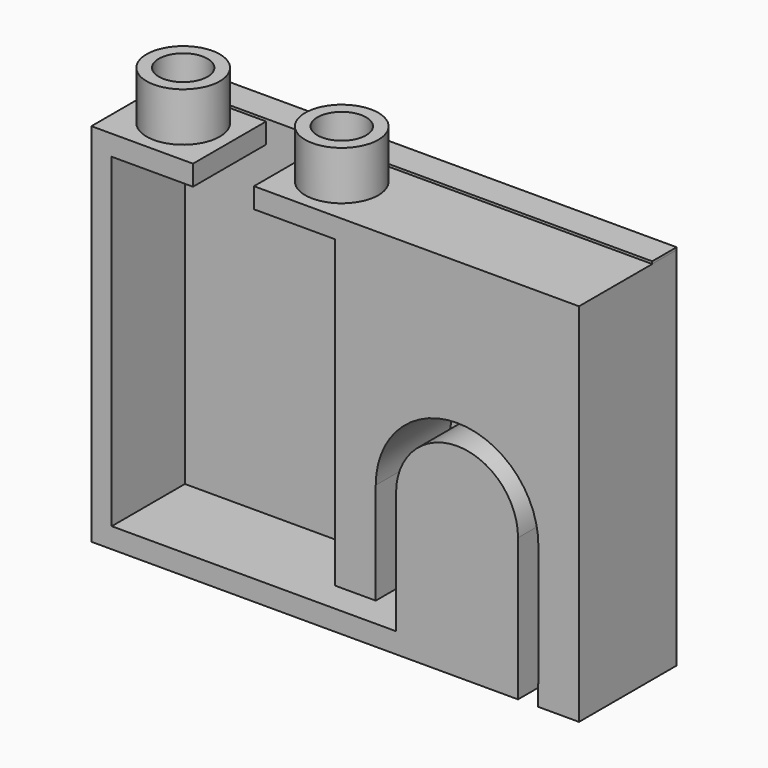
from build123d import *

# Parameters (mm, degrees)
F1_DEPTH = 15.875
F0_W     = 2.6458333332
F0_H     = 42.3358732487
F2_W     = 63.5
F2_H     = 47.625
F2_R     = 3.175
F3_DEPTH = 3.96875
F4_DEPTH = 6.35
F5_R     = 4.7625
F5_R_2   = 3.175
F6_DEPTH = 6.35
F7_R     = 3.175
F8_DEPTH = 25.4


# Not quite as in the source:
# - a feature names something its author has since deleted; it is built from what else it names


with BuildPart() as f1:
    # F0 (on Front) → F1 (new body)
    with BuildSketch(Plane.XZ):
        with BuildLine():
            Line((0, 44.979166582), (-31.75, 44.979166582))
            Line((-31.75, 44.979166582), (-31.75, 42.3358732487))
            Line((-31.75, 42.3358732487), (-31.75, 2.6458333332))
            Line((-31.75, 2.6458333332), (-26.4583333333, 2.6458333332))
            Line((-26.4583333333, 2.6458333332), (-26.4583333333, 15.875))
            ThreePointArc((-26.4583333333, 15.875), (-15.875, 26.4583333333), (-5.2916666667, 15.875))
            Line((-5.2916666667, 15.875), (-5.2916666667, 0))
            Line((-5.2916666667, 0), (0, 0))
            Line((0, 0), (0, 44.979166582))
        make_face()
        Polygon((0, -2.6458333333), (0, 0), (-5.2916666667, 0), (-5.309548229, 0), (-5.309548229, -2.6458333333), align=None)
        Polygon((-31.75, 42.3358732487), (-31.75, 44.979166582), (-34.3958333316, 44.979166582), (-37.0416664956, 44.979166582), (-42.3110765377, 44.979166582), (-42.3110765377, 42.3358732487), (-37.0416664956, 42.3358732487), (-34.3958333316, 42.3358732487), align=None)
    extrude(amount=F1_DEPTH)


with BuildPart() as f1b:
    # F0 (on Front) → F1, piece 2 (new body)
    with BuildSketch(Plane.XZ):
        with BuildLine():
            Line((-23.8125, 0), (-7.9375, 0))
            Line((-7.9375, 0), (-7.9375, 15.875))
            ThreePointArc((-7.9375, 15.875), (-15.875, 23.8125), (-23.8125, 15.875))
            Line((-23.8125, 15.875), (-23.8125, 0))
        make_face()
        Polygon((-26.4583333333, 0), (-31.75, 0), (-60.8213265341, 0), (-63.4671598673, 0), (-63.4671598673, -2.6458333333), (-7.9375, -2.6458333333), (-7.9375, 0), (-23.8125, 0), align=None)
        with Locations((-62.1442432007, 21.1679366243)):
            Rectangle(F0_W, F0_H)
        Polygon((-50.2485765377, 42.3358732487), (-50.2485765377, 44.979166582), (-55.5296598693, 44.979166582), (-58.175493201, 44.979166582), (-63.4671598673, 44.979166582), (-63.4671598673, 42.3358732487), (-60.8213265341, 42.3358732487), (-58.175493201, 42.3358732487), (-55.5296598693, 42.3358732487), align=None)
    extrude(amount=F1_DEPTH)


with BuildPart() as f3:
    # F2 (on Front) → F3 (new body)
    with BuildSketch(Plane.XZ):
        with Locations((-31.75, 21.4839725468)):
            Rectangle(F2_W, F2_H)
        with Locations((-53.975, 7.1964725468)):
            Circle(F2_R, mode=Mode.SUBTRACT)
        with Locations((-9.525, 7.1964725468)):
            Circle(F2_R, mode=Mode.SUBTRACT)
        with Locations((-52.284011212, 35.7714725468)):
            Circle(F2_R, mode=Mode.SUBTRACT)
        with Locations((-9.525, 35.7714725468)):
            Circle(F2_R, mode=Mode.SUBTRACT)
        with Locations((-52.284011212, 35.7714725468)):
            Circle(F2_R)
        with Locations((-53.975, 7.1964725468)):
            Circle(F2_R)
        with Locations((-9.525, 7.1964725468)):
            Circle(F2_R)
        with Locations((-9.525, 35.7714725468)):
            Circle(F2_R)
    extrude(amount=F3_DEPTH)


with BuildPart() as f4:
    # F2 (on Front) → F4 (new body)
    with BuildSketch(Plane.XZ):
        with Locations((-9.525, 35.7714725468)):
            Circle(F2_R)
    extrude(amount=-F4_DEPTH)


with BuildPart() as f4b:
    # F2 (on Front) → F4, piece 2 (new body)
    with BuildSketch(Plane.XZ):
        with Locations((-52.284011212, 35.7714725468)):
            Circle(F2_R)
    extrude(amount=-F4_DEPTH)


with BuildPart() as f4c:
    # F2 (on Front) → F4, piece 3 (new body)
    with BuildSketch(Plane.XZ):
        with Locations((-9.525, 7.1964725468)):
            Circle(F2_R)
    extrude(amount=-F4_DEPTH)


with BuildPart() as f4d:
    # F2 (on Front) → F4, piece 4 (new body)
    with BuildSketch(Plane.XZ):
        with Locations((-53.975, 7.1964725468)):
            Circle(F2_R)
    extrude(amount=-F4_DEPTH)


with BuildPart() as f6:
    # F5 (on face) → F6 (new body)
    with BuildSketch(Plane.XY.offset(44.979166582)):
        with Locations((-56.5985765377, -9.525)):
            Circle(F5_R)
        with Locations((-56.5985765377, -9.525)):
            Circle(F5_R_2, mode=Mode.SUBTRACT)
    extrude(amount=F6_DEPTH)


with BuildPart() as f6b:
    # F5 (on face) → F6, piece 2 (new body)
    with BuildSketch(Plane.XY.offset(44.979166582)):
        with Locations((-35.9610765377, -9.525)):
            Circle(F5_R)
        with Locations((-35.9610765377, -9.525)):
            Circle(F5_R_2, mode=Mode.SUBTRACT)
    extrude(amount=F6_DEPTH)


with BuildPart() as f8_tool:
    # F7 (on face) → F8 (new body)
    with BuildSketch(Plane.XY.offset(44.979166582)):
        with Locations((-35.9610765377, -9.525)):
            Circle(F7_R)
        with Locations((-56.5985765377, -9.525)):
            Circle(F7_R)
    extrude(amount=-F8_DEPTH)


with BuildPart() as f1_1:
    add(f1.part)

    # F8: cut by f8_tool
    add(f8_tool.part, mode=Mode.SUBTRACT)


with BuildPart() as f1b_1:
    add(f1b.part)

    # F8: cut by f8_tool
    add(f8_tool.part, mode=Mode.SUBTRACT)


solid = Compound([f3.part, f4.part, f4b.part, f4c.part, f4d.part, f6.part, f6b.part, f1_1.part, f1b_1.part])
